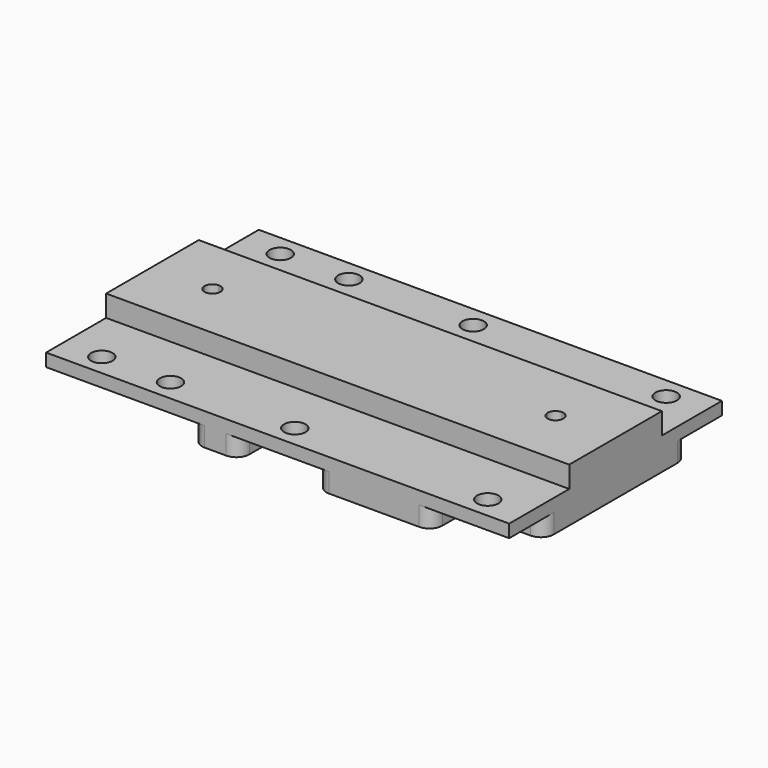
from build123d import *

# Parameters (mm, degrees)
F0_W     = 11
F0_H     = 10
F0_W_2   = 34
F0_H_2   = 42
F0_W_3   = 18
F0_W_4   = 27
F1_DEPTH = 4.5
F2_R     = 3
F4_DEPTH = 3
F6_DEPTH = 5
F7_DEPTH = 7.5
F8_DEPTH = 7.5


with BuildPart() as f1:
    # F0 (on Top) → F1 (new body)
    with BuildSketch(Plane.XY):
        with Locations((-25.173913, 37.042781)):
            Rectangle(F0_W, F0_H)
        with Locations((-47.673913, 11.042781)):
            Rectangle(F0_W_2, F0_H_2)
        with Locations((-25.173913, 11.042781)):
            Rectangle(F0_W, F0_H_2)
        with Locations((-10.673913, 11.042781)):
            Rectangle(F0_W_3, F0_H_2)
        with Locations((-25.173913, -14.957219)):
            Rectangle(F0_W, F0_H)
        with Locations((11.826087, 37.042781)):
            Rectangle(F0_W_4, F0_H)
        with Locations((11.826087, 11.042781)):
            Rectangle(F0_W_4, F0_H_2)
        with Locations((34.326087, 11.042781)):
            Rectangle(F0_W_3, F0_H_2)
        with Locations((11.826087, -14.957219)):
            Rectangle(F0_W_4, F0_H)
    extrude(amount=F1_DEPTH)

    # F2
    f2_edges = [f1.edges().sort_by_distance(p)[0] for p in [
        (-64.673913, 32.042781, 2.25),
        (-30.673913, 42.042781, 2.25),
        (-19.673913, 42.042781, 2.25),
        (-1.673913, 42.042781, 2.25),
        (25.326087, 42.042781, 2.25),
        (-1.673913, 32.042781, 2.25),
        (-19.673913, 32.042781, 2.25),
        (25.326087, 32.042781, 2.25),
        (43.326087, 32.042781, 2.25),
        (43.326087, -9.957219, 2.25),
        (25.326087, -9.957219, 2.25),
        (25.326087, -19.957219, 2.25),
        (-1.673913, -19.957219, 2.25),
        (-1.673913, -9.957219, 2.25),
        (-19.673913, -9.957219, 2.25),
        (-19.673913, -19.957219, 2.25),
        (-30.673913, -19.957219, 2.25),
        (-30.673913, -9.957219, 2.25),
        (-64.673913, -9.957219, 2.25),
        (-30.673913, 32.042781, 2.25),
    ]]
    fillet(f2_edges, radius=F2_R)

    # F3 (on face) → F4 (join)
    with BuildSketch(Plane.XY.offset(4.5)):
        Polygon((43.326087, 42.042781), (-64.673913, 42.042781), (-64.673913, 37.042781), (-64.673913, -14.957219), (-64.673913, -19.957219), (43.326087, -19.957219), (43.326087, -14.957219), (43.326087, 37.042781), align=None)
        with BuildLine():
            ThreePointArc((-53.173913, -14.957219), (-55.673913, -17.457219), (-58.173913, -14.957219))
            ThreePointArc((-58.173913, -14.957219), (-55.673913, -12.457219), (-53.173913, -14.957219))
        make_face(mode=Mode.SUBTRACT)
        with BuildLine():
            ThreePointArc((-37.173913, -14.957219), (-39.673913, -17.457219), (-42.173913, -14.957219))
            ThreePointArc((-42.173913, -14.957219), (-39.673913, -12.457219), (-37.173913, -14.957219))
        make_face(mode=Mode.SUBTRACT)
        with BuildLine():
            ThreePointArc((-8.173913, -14.957219), (-10.673913, -17.457219), (-13.173913, -14.957219))
            ThreePointArc((-13.173913, -14.957219), (-10.673913, -12.457219), (-8.173913, -14.957219))
        make_face(mode=Mode.SUBTRACT)
        with BuildLine():
            ThreePointArc((31.826087, -14.957219), (34.326087, -12.457219), (36.826087, -14.957219))
            ThreePointArc((36.826087, -14.957219), (34.326087, -17.457219), (31.826087, -14.957219))
        make_face(mode=Mode.SUBTRACT)
        with BuildLine():
            ThreePointArc((-53.173913, 37.042781), (-55.673913, 34.542781), (-58.173913, 37.042781))
            ThreePointArc((-58.173913, 37.042781), (-55.673913, 39.542781), (-53.173913, 37.042781))
        make_face(mode=Mode.SUBTRACT)
        with BuildLine():
            ThreePointArc((-37.173913, 37.042781), (-39.673913, 34.542781), (-42.173913, 37.042781))
            ThreePointArc((-42.173913, 37.042781), (-39.673913, 39.542781), (-37.173913, 37.042781))
        make_face(mode=Mode.SUBTRACT)
        with BuildLine():
            ThreePointArc((-8.173913, 37.042781), (-10.673913, 34.542781), (-13.173913, 37.042781))
            ThreePointArc((-13.173913, 37.042781), (-10.673913, 39.542781), (-8.173913, 37.042781))
        make_face(mode=Mode.SUBTRACT)
        with BuildLine():
            ThreePointArc((31.826087, 37.042781), (34.326087, 39.542781), (36.826087, 37.042781))
            ThreePointArc((36.826087, 37.042781), (34.326087, 34.542781), (31.826087, 37.042781))
        make_face(mode=Mode.SUBTRACT)
    extrude(amount=F4_DEPTH)

    # F5 (on face) → F6 (join)
    with BuildSketch(Plane.XY.offset(7.5)):
        with BuildLine():
            Line((-50.673913, 24.542781), (-64.673913, 24.542781))
            Line((-64.673913, 24.542781), (-64.673913, 11.042781))
            Line((-64.673913, 11.042781), (-52.523913, 11.042781))
            ThreePointArc((-52.523913, 11.042781), (-51.982061, 12.350929), (-50.673913, 12.892781))
            Line((-50.673913, 12.892781), (-50.673913, 24.542781))
        make_face()
        with BuildLine():
            Line((29.326087, 24.542781), (-50.673913, 24.542781))
            Line((-50.673913, 24.542781), (-50.673913, 12.892781))
            ThreePointArc((-50.673913, 12.892781), (-49.365766, 12.350929), (-48.823913, 11.042781))
            Line((-48.823913, 11.042781), (27.476087, 11.042781))
            ThreePointArc((27.476087, 11.042781), (28.017939, 12.350929), (29.326087, 12.892781))
            Line((29.326087, 12.892781), (29.326087, 24.542781))
        make_face()
        with BuildLine():
            Line((-52.523913, 11.042781), (-64.673913, 11.042781))
            Line((-64.673913, 11.042781), (-64.673913, -2.457219))
            Line((-64.673913, -2.457219), (-50.673913, -2.457219))
            Line((-50.673913, -2.457219), (-50.673913, 9.192781))
            ThreePointArc((-50.673913, 9.192781), (-51.982061, 9.734634), (-52.523913, 11.042781))
        make_face()
        with BuildLine():
            Line((43.326087, 24.542781), (29.326087, 24.542781))
            Line((29.326087, 24.542781), (29.326087, 12.892781))
            ThreePointArc((29.326087, 12.892781), (30.634234, 12.350929), (31.176087, 11.042781))
            Line((31.176087, 11.042781), (43.326087, 11.042781))
            Line((43.326087, 11.042781), (43.326087, 24.542781))
        make_face()
        with BuildLine():
            Line((27.476087, 11.042781), (-48.823913, 11.042781))
            ThreePointArc((-48.823913, 11.042781), (-49.365766, 9.734634), (-50.673913, 9.192781))
            Line((-50.673913, 9.192781), (-50.673913, -2.457219))
            Line((-50.673913, -2.457219), (29.326087, -2.457219))
            Line((29.326087, -2.457219), (29.326087, 9.192781))
            ThreePointArc((29.326087, 9.192781), (28.017939, 9.734634), (27.476087, 11.042781))
        make_face()
        with BuildLine():
            Line((43.326087, -2.457219), (43.326087, 11.042781))
            Line((43.326087, 11.042781), (31.176087, 11.042781))
            ThreePointArc((31.176087, 11.042781), (30.634234, 9.734634), (29.326087, 9.192781))
            Line((29.326087, 9.192781), (29.326087, -2.457219))
            Line((29.326087, -2.457219), (43.326087, -2.457219))
        make_face()
    extrude(amount=F6_DEPTH)

    # F7 (cut): a face of the model
    f7_faces = [f1.faces().sort_by_distance(p)[0] for p in [
        (-50.673913, 11.042781, 7.5),
    ]]
    extrude(f7_faces, amount=-F7_DEPTH, mode=Mode.SUBTRACT)

    # F8 (cut): a face of the model
    f8_faces = [f1.faces().sort_by_distance(p)[0] for p in [
        (29.326087, 11.042781, 7.5),
    ]]
    extrude(f8_faces, amount=-F8_DEPTH, mode=Mode.SUBTRACT)


solid = f1.part
